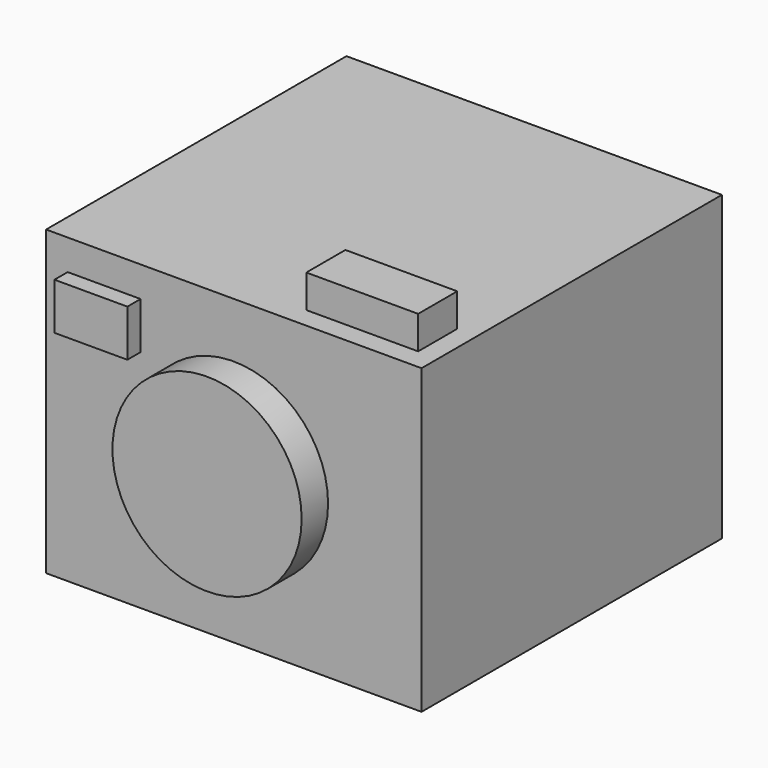
from build123d import *

# Parameters (mm, degrees)
F0_W      = 113.6225089431
F0_H      = 91.5519557893
F1_DEPTH  = 113.62251
F2_R      = 28.629575464
F3_DEPTH  = 10
F4_DEPTH  = 18
F7_W      = 33.8436812162
F7_H      = 14.7902220488
F8_DEPTH  = 10
F9_W      = 22.0619104803
F9_H      = 14.1544528306
F10_DEPTH = 5
F11_W     = 113.6225089431
F11_H     = 91.5519557893
F12_DEPTH = 60


# Not quite as in the source:
# - the program builds the solid bodies; features that only make, move or delete a surface that nothing else refers to are left out


with BuildPart() as f1:
    # F0 (on Front) → F1 (new body)
    with BuildSketch(Plane.XZ):
        with Locations((0.1021772623, -0.4832614213)):
            Rectangle(F0_W, F0_H)
    extrude(amount=F1_DEPTH)

    # F2 (on face) → F3 (join)
    with BuildSketch(Plane.XZ.offset(113.62251)):
        Circle(F2_R)
    extrude(amount=F3_DEPTH)

    # F4 (add): a face of the model
    f4_faces = [f1.faces().sort_by_distance(p)[0] for p in [
        (0, -123.62251, 0),
    ]]
    extrude(f4_faces, amount=-F4_DEPTH)

    # F7 (on face) → F8 (join)
    with BuildSketch(Plane.XY.offset(45.2927164733)):
        with Locations((33.9821465313, -100.0008359551)):
            Rectangle(F7_W, F7_H)
    extrude(amount=F8_DEPTH)

    # F9 (on face) → F10 (join)
    with BuildSketch(Plane.XZ.offset(113.62251)):
        with Locations((-39.1396004707, 29.0038492531)):
            Rectangle(F9_W, F9_H)
    extrude(amount=F10_DEPTH)

    # F11 (on face) → F12 (join)
    with BuildSketch(Plane(origin=(0, 0, 0), x_dir=(-1, 0, 0), z_dir=(0, 1, 0))):
        with Locations((-0.1021772623, -0.4832614213)):
            Rectangle(F11_W, F11_H)
    extrude(amount=-F12_DEPTH)


solid = f1.part
